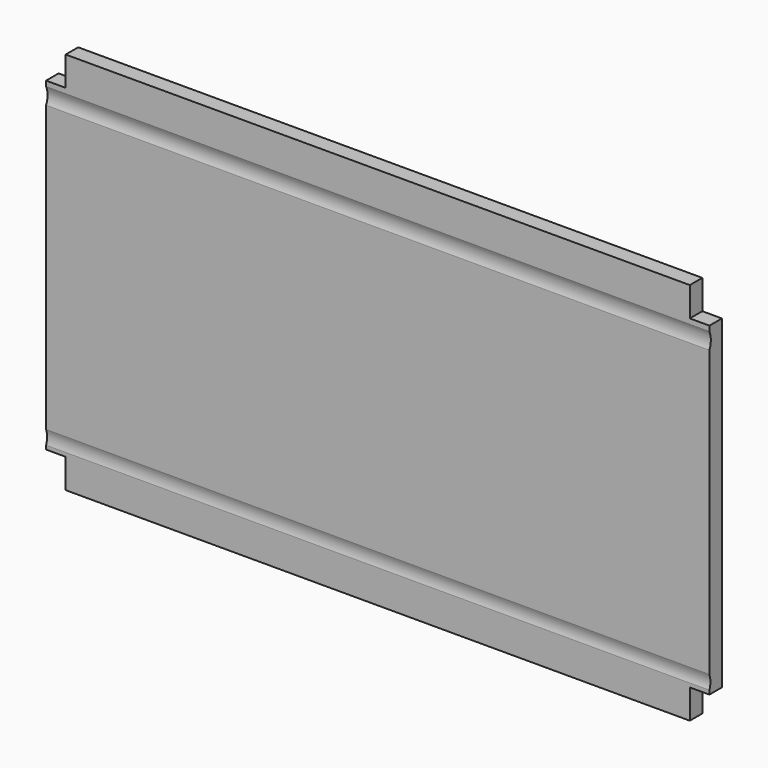
from build123d import *

# Parameters (mm, degrees)
F0_W     = 1695
F0_H     = 980
F1_DEPTH = 40
F2_R     = 50
F3_DEPTH = 1695.001
F6_W     = 40
F6_H     = 75
F7_DEPTH = 50
F8_W     = 40
F8_H     = 75
F9_DEPTH = 50


# Not quite as in the source:
# - a feature of the source that left no trace in its solid (it failed there, or was rolled back) is left out


with BuildPart() as f1:
    # F0 (on Front) → F1 (new body)
    with BuildSketch(Plane.XZ):
        with Locations((847.5, -490)):
            Rectangle(F0_W, F0_H)
    extrude(amount=F1_DEPTH)

    # F2 (on face) → F3 (cut, through all)
    with BuildSketch(Plane(origin=(0, 0, 0), x_dir=(0, -1, 0), z_dir=(-1, 0, 0))):
        with Locations((85.3642523289, -109.1325581074)):
            Circle(F2_R)
        with Locations((86.7706388235, -877.3503899574)):
            Circle(F2_R)
    extrude(amount=-F3_DEPTH, mode=Mode.SUBTRACT)

    # F6 (on face) → F7 (cut)
    with BuildSketch(Plane(origin=(0, 0, 0), x_dir=(0, -1, 0), z_dir=(-1, 0, 0))):
        with Locations((20, -37.5)):
            Rectangle(F6_W, F6_H)
        with Locations((20, -942.5)):
            Rectangle(F6_W, F6_H)
    extrude(amount=-F7_DEPTH, mode=Mode.SUBTRACT)

    # F8 (on face) → F9 (cut)
    with BuildSketch(Plane.YZ.offset(1695)):
        with Locations((-20, -37.5)):
            Rectangle(F8_W, F8_H)
        with Locations((-20, -942.5)):
            Rectangle(F8_W, F8_H)
    extrude(amount=-F9_DEPTH, mode=Mode.SUBTRACT)


solid = f1.part
